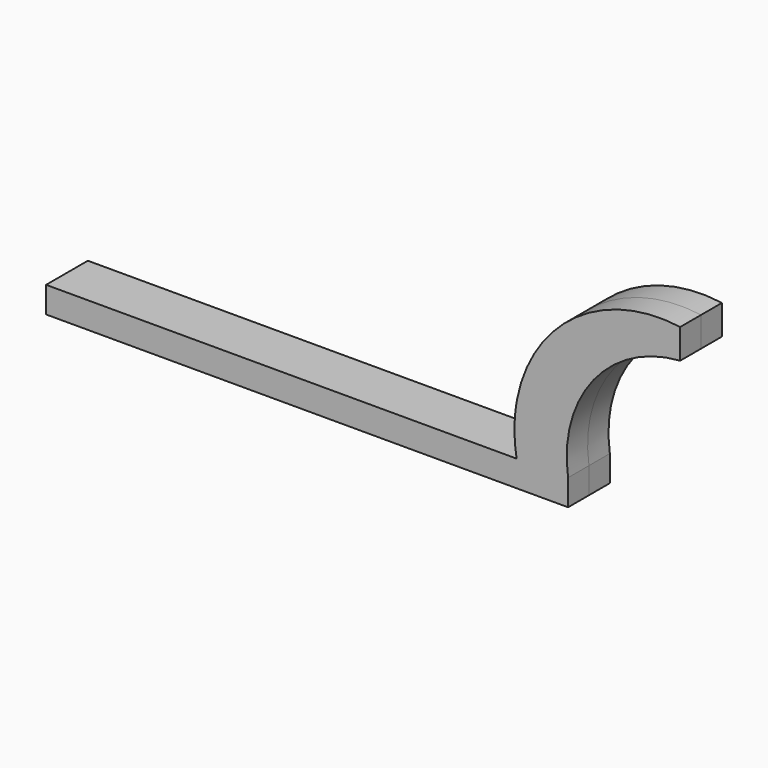
from build123d import *

# Parameters (mm, degrees)
F4_DEPTH = 53.34


# Not quite as in the source:
# - the program builds the solid bodies; features that only make, move or delete a surface that nothing else refers to are left out


with BuildPart() as f4:
    # F0 (on Front) → F4 (new body, symmetric)
    with BuildSketch(Plane.XZ):
        with BuildLine():
            Line((-548.9229032603, 53.3517466559), (-548.9229032603, 0))
            Line((-548.9229032603, 0), (517.8770967397, 0))
            Line((517.8770967397, 0), (517.8770967397, 53.3517466559))
            ThreePointArc((517.8770967397, 53.3517466559), (569.8826534338, 246.0368993204), (746.9217918528, 338.1742394829))
            Line((746.9217918528, 338.1742394829), (746.9217918528, 398.8678294032))
            ThreePointArc((746.9217918528, 398.8678294032), (533.7351343449, 346.9515616778), (414.162291011, 162.9782349944))
            ThreePointArc((414.162291011, 162.9782349944), (410.443214336, 139.7945515932), (408.564564689, 116.3897362155))
            ThreePointArc((408.564564689, 116.3897362155), (408.9628088542, 84.760149458), (412.718017276, 53.3517466559))
            Line((412.718017276, 53.3517466559), (111.3264834418, 53.3517466559))
            Line((111.3264834418, 53.3517466559), (78.2992156876, 53.3517466559))
            Line((78.2992156876, 53.3517466559), (0, 53.3517466559))
            Line((0, 53.3517466559), (-548.9229032603, 53.3517466559))
        make_face()
    extrude(amount=F4_DEPTH, both=True)


solid = f4.part
